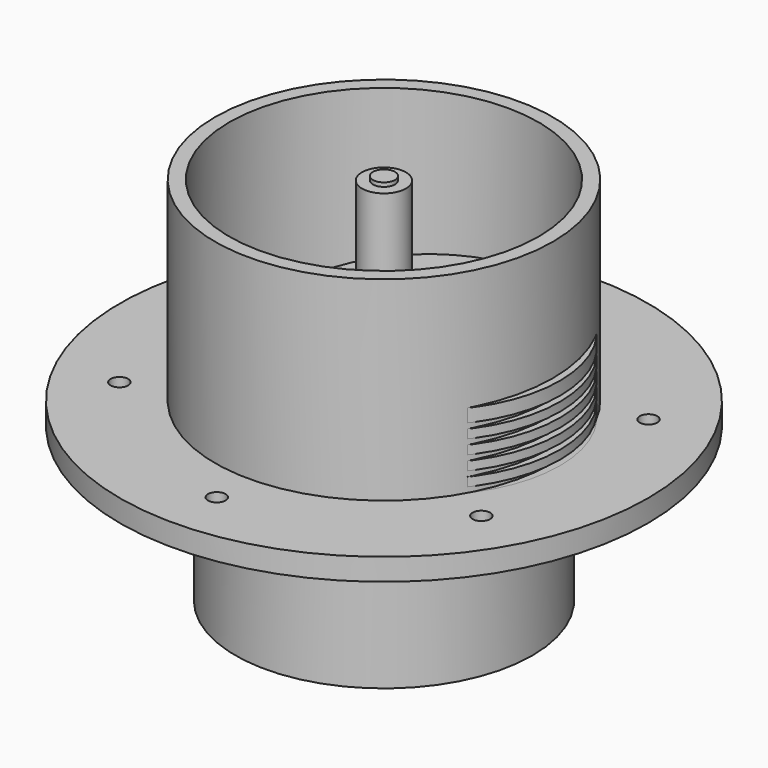
from build123d import *

# Parameters (mm, degrees)
F0_R      = 60
F0_R_2    = 2
F1_DEPTH  = 5
F2_R      = 38.5
F2_R_2    = 35
F3_DEPTH  = 2.5
F4_R      = 38.5
F4_R_2    = 35
F5_DEPTH  = 1.5
F6_R      = 38.4
F6_R_2    = 35.18
F7_DEPTH  = 49.3
F8_R      = 5
F9_DEPTH  = 49.1
F10_R     = 2
F11_DEPTH = 15
F12_R     = 2
F13_DEPTH = 15
F14_R     = 33.75
F14_R_2   = 2
F15_DEPTH = 35
F16_R     = 60
F16_R_2   = 2
F16_R_3   = 2.75
F16_R_4   = 4
F17_DEPTH = 5
F18_R     = 38.5
F18_R_2   = 35
F19_DEPTH = 3
F20_R     = 2
F21_DEPTH = 49.301
F24_R     = 2.5
F25_DEPTH = 50


with BuildPart() as f1:
    # F0 (on Top) → F1 (new body)
    with BuildSketch(Plane.XY):
        Circle(F0_R)
        with Locations((-41.1362066798, -23.75)):
            Circle(F0_R_2, mode=Mode.SUBTRACT)
        with Locations((0, -47.5)):
            Circle(F0_R_2, mode=Mode.SUBTRACT)
        with Locations((41.1362066798, -23.75)):
            Circle(F0_R_2, mode=Mode.SUBTRACT)
        with Locations((-41.1362066798, 23.75)):
            Circle(F0_R_2, mode=Mode.SUBTRACT)
        with Locations((41.1362066798, 23.75)):
            Circle(F0_R_2, mode=Mode.SUBTRACT)
        with Locations((0, 47.5)):
            Circle(F0_R_2, mode=Mode.SUBTRACT)
    extrude(amount=F1_DEPTH)

    # F2 (on face) → F3 (cut)
    with BuildSketch(Plane.XY.offset(5)):
        Circle(F2_R)
        Circle(F2_R_2, mode=Mode.SUBTRACT)
    extrude(amount=-F3_DEPTH, mode=Mode.SUBTRACT)


with BuildPart() as f5:
    # F4 (on Top) → F5 (new body)
    with BuildSketch(Plane.XY):
        Circle(F4_R)
        Circle(F4_R_2, mode=Mode.SUBTRACT)
    extrude(amount=F5_DEPTH)


with BuildPart() as f7:
    # F6 (on Top) → F7 (new body)
    with BuildSketch(Plane.XY):
        Circle(F6_R)
        Circle(F6_R_2, mode=Mode.SUBTRACT)
    extrude(amount=F7_DEPTH)


with BuildPart() as f9:
    # F8 (on Top) → F9 (new body)
    with BuildSketch(Plane.XY):
        Circle(F8_R)
    extrude(amount=F9_DEPTH)

    # F10 (on face) → F11 (cut)
    with BuildSketch(Plane.XY.offset(49.1)):
        Circle(F10_R)
    extrude(amount=-F11_DEPTH, mode=Mode.SUBTRACT)

    # F12 (on face) → F13 (cut)
    with BuildSketch(Plane(origin=(0, 0, 0), x_dir=(1, 0, 0), z_dir=(0, 0, -1))):
        Circle(F12_R)
    extrude(amount=-F13_DEPTH, mode=Mode.SUBTRACT)


with BuildPart() as f15:
    # F14 (on Top) → F15 (new body)
    with BuildSketch(Plane.XY):
        Circle(F14_R)
        Circle(F14_R_2, mode=Mode.SUBTRACT)
    extrude(amount=-F15_DEPTH)


with BuildPart() as f17:
    # F16 (on Top) → F17 (new body)
    with BuildSketch(Plane.XY):
        Circle(F16_R)
        with Locations((-41.1362066798, -23.75)):
            Circle(F16_R_2, mode=Mode.SUBTRACT)
        with Locations((0, -47.5)):
            Circle(F16_R_2, mode=Mode.SUBTRACT)
        with Locations((41.1362066798, -23.75)):
            Circle(F16_R_2, mode=Mode.SUBTRACT)
        with Locations((-41.1362066798, 23.75)):
            Circle(F16_R_2, mode=Mode.SUBTRACT)
        Circle(F16_R_3, mode=Mode.SUBTRACT)
        with Locations((22, 0)):
            Circle(F16_R_4, mode=Mode.SUBTRACT)
        with Locations((41.1362066798, 23.75)):
            Circle(F16_R_2, mode=Mode.SUBTRACT)
        with Locations((0, 47.5)):
            Circle(F16_R_2, mode=Mode.SUBTRACT)
    extrude(amount=F17_DEPTH)

    # F18 (on face) → F19 (cut)
    with BuildSketch(Plane(origin=(0, 0, 0), x_dir=(1, 0, 0), z_dir=(0, 0, -1))):
        Circle(F18_R)
        Circle(F18_R_2, mode=Mode.SUBTRACT)
    extrude(amount=-F19_DEPTH, mode=Mode.SUBTRACT)

    # F20 (on face) → F21 (cut, through all)
    with BuildSketch(Plane(origin=(0, 0, 0), x_dir=(1, 0, 0), z_dir=(0, 0, -1))):
        with Locations((10, 9)):
            Circle(F20_R)
        with Locations((10, -9)):
            Circle(F20_R)
    extrude(amount=-F21_DEPTH, mode=Mode.SUBTRACT)


with BuildPart() as f23:
    # F22 (on Front) → F23 (revolve)
    with BuildSketch(Plane.XZ):
        Polygon((10, 22), (10, 0), (40, 0), (40, 5), (34, 5), (34, 6.2), (40, 6.2), (40, 8.2), (34, 8.2), (34, 9.4), (40, 9.4), (40, 11.4), (34, 11.4), (34, 12.6), (40, 12.6), (40, 14.6), (34, 14.6), (34, 15.8), (40, 15.8), (40, 17.8), (34, 17.8), (34, 19), (40, 19), (40, 22), align=None)
    revolve(axis=Axis((10, 0, 11), (0, 0, -1)))


with BuildPart() as f25:
    # F24 (on Top) → F25 (new body)
    with BuildSketch(Plane.XY):
        Circle(F24_R)
    extrude(amount=F25_DEPTH)


solid = Compound([f1.part, f5.part, f7.part, f9.part, f15.part, f17.part, f23.part, f25.part])
